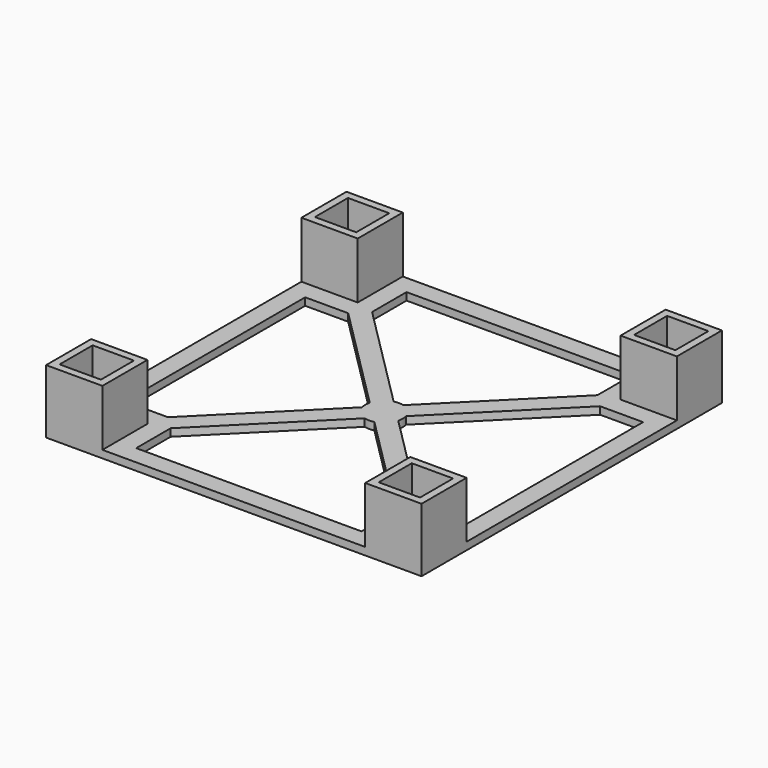
from build123d import *

# Parameters (mm, degrees)
F0_W        = 100
F0_H        = 100
F1_DEPTH    = 2
F2_W        = 15
F2_H        = 15
F3_DEPTH    = 15
F4_T        = 2
F4_T3_DEPTH = 19
F4_T5_DEPTH = 19
F4_T7_DEPTH = 19
F4_T9_DEPTH = 19
F6_DEPTH    = 2.001


# Not quite as in the source:
# - a shell that OpenCascade refuses in one call is made with other operations: the cavity is built on its own and cut out


with BuildPart() as f1:
    # F0 (on Top) → F1 (new body)
    with BuildSketch(Plane.XY):
        Rectangle(F0_W, F0_H)
    extrude(amount=F1_DEPTH)

    # F2 (on face) → F3 (join)
    with BuildSketch(Plane.XY.offset(2)):
        with Locations((-42.5, -42.5)):
            Rectangle(F2_W, F2_H)
        with Locations((-42.5, 42.5)):
            Rectangle(F2_W, F2_H)
        with Locations((42.5, 42.5)):
            Rectangle(F2_W, F2_H)
        with Locations((42.5, -42.5)):
            Rectangle(F2_W, F2_H)
    extrude(amount=F3_DEPTH)

    # F4: shell of thickness 2, made by hand


with BuildPart() as f4_core1:
    # F4_t2: copy of F1
    add(f1.part)

    # the walls: a layer under each face that stays
    f4_faces = [f4_core1.faces().sort_by_distance(p)[0] for p in [
        (50, -42.8571428571, 15.7857142857),
        (0, 0, 0),
        (-50, 42.8571428571, 15.7857142857),
        (-35, -42.5, 9.5),
        (-42.5, -35, 9.5),
        (-42.5, 35, 9.5),
        (-35, 42.5, 9.5),
        (42.8571428571, 50, 15.7857142857),
        (35, 42.5, 9.5),
        (42.5, 35, 9.5),
        (0, 0, 2),
        (35, -42.5, 9.5),
        (42.5, -35, 9.5),
        (-42.8571428571, -50, 15.7857142857),
    ]]
    thicken(f4_faces, amount=-F4_T, mode=Mode.SUBTRACT)

    # F4_s4 → F4_t3 (cut)
    with BuildSketch(Plane.XZ.offset(33)):
        Polygon((-34.98, 2.02), (-37, 2), (-37, 0), (-35, 0), align=None)
        Polygon((34.98, 2.02), (35, 0), (37, 0), (37, 2), align=None)
    extrude(amount=F4_T3_DEPTH, mode=Mode.SUBTRACT)

    # F4_s6 → F4_t5 (cut)
    with BuildSketch(Plane.YZ.offset(-52)):
        Polygon((-34.98, 2.02), (-37, 2), (-37, 0), (-35, 0), align=None)
        Polygon((34.98, 2.02), (37, 2), (37, 0), (35, 0), align=None)
    extrude(amount=F4_T5_DEPTH, mode=Mode.SUBTRACT)

    # F4_s8 → F4_t7 (cut)
    with BuildSketch(Plane.XZ.offset(-52)):
        Polygon((-34.98, 2.02), (-37, 2), (-37, 0), (-35, 0), align=None)
        Polygon((34.98, 2.02), (37, 2), (37, 0), (35, 0), align=None)
    extrude(amount=F4_T7_DEPTH, mode=Mode.SUBTRACT)

    # F4_s10 → F4_t9 (cut)
    with BuildSketch(Plane.YZ.offset(33)):
        Polygon((34.98, 2.02), (37, 2), (37, 0), (35, 0), align=None)
        Polygon((-34.98, 2.02), (-35, 0), (-37, 0), (-37, 2), align=None)
    extrude(amount=F4_T9_DEPTH, mode=Mode.SUBTRACT)


with BuildPart() as f1_1:
    add(f1.part)

    # what is left inside the walls is the cavity
    f4_cavity = [f4_core1.part.solids().sort_by_distance(p)[0] for p in [
        (47.98, -42.5, 12),
        (47.98, 42.5, 12),
        (-42.5, -47.98, 12),
        (-37.02, 42.5, 12),
    ]]
    add(f4_cavity, mode=Mode.SUBTRACT)

    # F5 (on face) → F6 (cut, through all)
    with BuildSketch(Plane.XY.offset(2)):
        with BuildLine():
            Line((-30.0000010431, -45.0000010431), (30.0000010431, -45.0000010431))
            Line((30.0000010431, -45.0000010431), (30.0000010431, -33.535534949))
            Line((30.0000010431, -33.535534949), (1.2940952255, -4.8296291314))
            ThreePointArc((1.2940952255, -4.8296291314), (0, -5), (-1.2940952255, -4.8296291314))
            Line((-1.2940952255, -4.8296291314), (-30.0000010431, -33.535534949))
            Line((-30.0000010431, -33.535534949), (-30.0000010431, -45.0000010431))
        make_face()
        with BuildLine():
            Line((-33.535534949, 30.0000010431), (-45.0000010431, 30.0000010431))
            Line((-45.0000010431, 30.0000010431), (-45.0000010431, -30.0000010431))
            Line((-45.0000010431, -30.0000010431), (-33.535534949, -30.0000010431))
            Line((-33.535534949, -30.0000010431), (-4.8296291314, -1.2940952255))
            ThreePointArc((-4.8296291314, -1.2940952255), (-5, 0), (-4.8296291314, 1.2940952255))
            Line((-4.8296291314, 1.2940952255), (-33.535534949, 30.0000010431))
        make_face()
        with BuildLine():
            Line((30.0000010431, 45.0000010431), (-30.0000010431, 45.0000010431))
            Line((-30.0000010431, 45.0000010431), (-30.0000010431, 33.535534949))
            Line((-30.0000010431, 33.535534949), (-1.2940952255, 4.8296291314))
            ThreePointArc((-1.2940952255, 4.8296291314), (0, 5), (1.2940952255, 4.8296291314))
            Line((1.2940952255, 4.8296291314), (30.0000010431, 33.535534949))
            Line((30.0000010431, 33.535534949), (30.0000010431, 45.0000010431))
        make_face()
        with BuildLine():
            Line((45.0000010431, -30.0000010431), (45.0000010431, 30.0000010431))
            Line((45.0000010431, 30.0000010431), (33.535534949, 30.0000010431))
            Line((33.535534949, 30.0000010431), (4.8296291314, 1.2940952255))
            ThreePointArc((4.8296291314, 1.2940952255), (5, 0), (4.8296291314, -1.2940952255))
            Line((4.8296291314, -1.2940952255), (33.535534949, -30.0000010431))
            Line((33.535534949, -30.0000010431), (45.0000010431, -30.0000010431))
        make_face()
    extrude(amount=-F6_DEPTH, mode=Mode.SUBTRACT)


solid = f1_1.part
